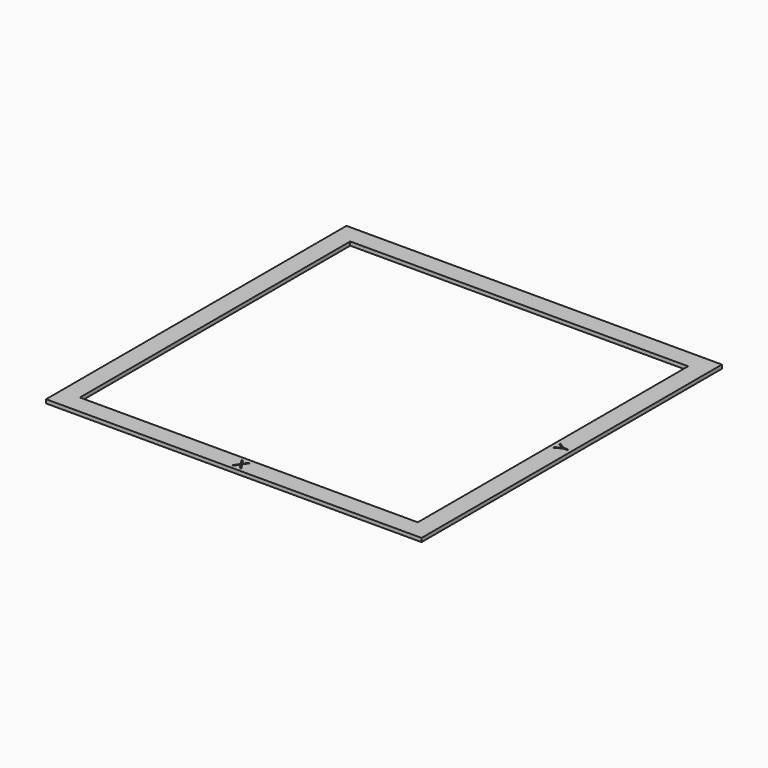
from build123d import *

# Parameters (mm, degrees)
F0_W         = 100
F0_H         = 100
F0_W_2       = 90
F0_H_2       = 90
F1_DEPTH     = 1
F2_TEXT_SIZE = 4.1666666667
F3_DEPTH     = 1.001


# Not quite as in the source:
# - Text() gives the source's letters only with a copy of the font that has no kerning and outlines rounded to 1/6400 em; it was checked with that copy


with BuildPart() as f1:
    # F0 (on Top) → F1 (new body)
    with BuildSketch(Plane.XY):
        with Locations((50, 50)):
            Rectangle(F0_W, F0_H)
        with Locations((50, 50)):
            Rectangle(F0_W_2, F0_H_2, mode=Mode.SUBTRACT)
    extrude(amount=F1_DEPTH)

    # F2 (on face) → F3 (cut, through all)
    with BuildSketch(Plane.XY.offset(1)):
        with Locations((48.8030729167, 1)):
            Text('X', F2_TEXT_SIZE, font='Open Sans', text_align=(TextAlign.LEFT, TextAlign.BOTTOM))
        with Locations(Location((99, 48.8332421875), (0, 0, 90))):
            Text('Y', F2_TEXT_SIZE, font='Open Sans', text_align=(TextAlign.LEFT, TextAlign.BOTTOM))
    extrude(amount=-F3_DEPTH, mode=Mode.SUBTRACT)


solid = f1.part
